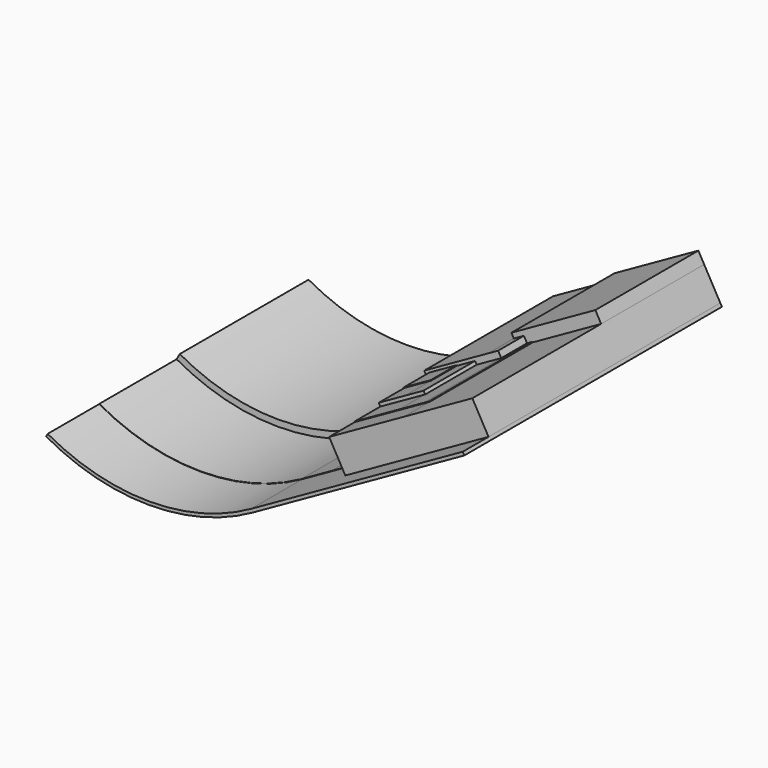
from build123d import *

# Parameters (mm, degrees)
F1_DEPTH = 100
F2_DEPTH = 90
F3_DEPTH = 80
F4_DEPTH = 80
F5_DEPTH = 70
F6_DEPTH = 60
F7_DEPTH = 50
F8_DEPTH = 40


with BuildPart() as f1:
    # F0 (on Front) → F1 (new body)
    with BuildSketch(Plane.XZ):
        with BuildLine():
            Line((50.8452397293, 26.2241268437), (29.5219979318, 14.223603626))
            ThreePointArc((29.5219979318, 14.223603626), (-2.0391196005, 5.9907088835), (-33.6008071966, 14.221417955))
            Line((-33.6008071966, 14.221417955), (-34.0891893351, 13.3487880868))
            ThreePointArc((-34.0891893351, 13.3487880868), (-2.0385061949, 4.9907089067), (30.0114505771, 13.3515729915))
            Line((30.0114505771, 13.3515729915), (95.813926037, 50.3845974272))
            Line((95.813926037, 50.3845974272), (95.3234723322, 51.2560646748))
            Line((95.3234723322, 51.2560646748), (50.8452397293, 26.2241268437))
        make_face()
    extrude(amount=F1_DEPTH)


with BuildPart() as f2:
    # F0 (on Front) → F2 (new body)
    with BuildSketch(Plane.XZ):
        Polygon((50.7948435843, 26.3136737049), (50.8452397293, 26.2241268437), (95.3234723322, 51.2560646748), (90.3044164077, 60.1742210862), (69.0536898036, 48.2145087485), (45.8261838048, 35.1422832552), (49.7882909537, 28.1021761505), align=None)
    extrude(amount=F2_DEPTH)


with BuildPart() as f3:
    # F0 (on Front) → F3 (new body)
    with BuildSketch(Plane.XZ):
        with BuildLine():
            ThreePointArc((-33.6008071966, 14.221417955), (-2.0391196005, 5.9907088835), (29.5219979318, 14.223603626))
            Line((29.5219979318, 14.223603626), (50.8452397293, 26.2241268437))
            Line((50.8452397293, 26.2241268437), (50.7948435843, 26.3136737049))
            Line((50.7948435843, 26.3136737049), (38.4987711206, 19.393557876))
            Line((38.4987711206, 19.393557876), (29.0659948309, 14.0848786448))
            ThreePointArc((29.0659948309, 14.0848786448), (-2.2719574378, 6.0911209367), (-33.5519689827, 14.3086809418))
            Line((-33.5519689827, 14.3086809418), (-33.6008071966, 14.221417955))
        make_face()
    extrude(amount=F3_DEPTH)


with BuildPart() as f4:
    # F0 (on Front) → F4 (new body)
    with BuildSketch(Plane.XZ):
        Polygon((45.8261838048, 35.1422832552), (69.0536898036, 48.2145087485), (68.9724342199, 48.3588884915), (67.2759677307, 47.4041328458), (59.6421667017, 43.1079002486), (45.7449282211, 35.2866629982), align=None)
    extrude(amount=F4_DEPTH)


with BuildPart() as f5:
    # F0 (on Front) → F5 (new body)
    with BuildSketch(Plane.XZ):
        Polygon((38.4987711206, 19.393557876), (50.7948435843, 26.3136737049), (49.7882909537, 28.1021761505), (43.2631740892, 24.5774321962), (37.4072678387, 21.4141830802), align=None)
    extrude(amount=F5_DEPTH)


with BuildPart() as f5b:
    # F0 (on Front) → F5, piece 2 (new body)
    with BuildSketch(Plane.XZ):
        Polygon((45.2470448009, 36.1713318051), (45.7449282211, 35.2866629982), (59.6421667017, 43.1079002486), (59.1442832815, 43.9925690556), (53.4865097086, 40.8084264301), align=None)
    extrude(amount=F5_DEPTH)


with BuildPart() as f6:
    # F0 (on Front) → F6 (new body)
    with BuildSketch(Plane.XZ):
        Polygon((43.2631740892, 24.5774321962), (49.7882909537, 28.1021761505), (45.8261838048, 35.1422832552), (45.7449282211, 35.2866629982), (45.2470448009, 36.1713318051), (53.4865097086, 40.8084264301), (53.4059276803, 40.95160936), (44.9516252368, 36.1936061575), (49.453318119, 28.1947311014), (43.1277044117, 24.8282179236), align=None)
    extrude(amount=F6_DEPTH)


with BuildPart() as f7:
    # F0 (on Front) → F7 (new body)
    with BuildSketch(Plane.XZ):
        with BuildLine():
            Line((-32.5752047057, 16.0539406781), (-33.5519689827, 14.3086809418))
            ThreePointArc((-33.5519689827, 14.3086809418), (-2.2719574378, 6.0911209367), (29.0659948309, 14.0848786448))
            Line((29.0659948309, 14.0848786448), (38.4987711206, 19.393557876))
            Line((38.4987711206, 19.393557876), (37.4072678387, 21.4141830802))
            Line((37.4072678387, 21.4141830802), (43.2631740892, 24.5774321962))
            Line((43.2631740892, 24.5774321962), (43.1277044117, 24.8282179236))
            Line((43.1277044117, 24.8282179236), (49.453318119, 28.1947311014))
            Line((49.453318119, 28.1947311014), (44.9516252368, 36.1936061575))
            Line((44.9516252368, 36.1936061575), (53.4059276803, 40.95160936))
            Line((53.4059276803, 40.95160936), (53.4865097086, 40.8084264301))
            Line((53.4865097086, 40.8084264301), (59.1442832815, 43.9925690556))
            Line((59.1442832815, 43.9925690556), (59.6421667017, 43.1079002486))
            Line((59.6421667017, 43.1079002486), (67.2759677307, 47.4041328458))
            Line((67.2759677307, 47.4041328458), (66.3095066613, 49.1213982263))
            Line((66.3095066613, 49.1213982263), (63.190689116, 47.3661565647))
            Line((63.190689116, 47.3661565647), (43.3571876206, 36.2040454072))
            Line((43.3571876206, 36.2040454072), (47.5722491088, 28.7144740215))
            Line((47.5722491088, 28.7144740215), (36.3952242818, 22.4241478499))
            Line((36.3952242818, 22.4241478499), (28.4962685386, 16.0560553203))
            ThreePointArc((28.4962685386, 16.0560553203), (-2.0391923145, 8.0907088823), (-32.5752047057, 16.0539406781))
        make_face()
    extrude(amount=F7_DEPTH)


with BuildPart() as f8:
    # F0 (on Front) → F8 (new body)
    with BuildSketch(Plane.XZ):
        Polygon((69.0536898036, 48.2145087485), (90.3044164077, 60.1742210862), (88.5034794178, 63.3742328025), (62.4374687791, 48.7045231575), (63.190689116, 47.3661565647), (66.3095066613, 49.1213982263), (67.2759677307, 47.4041328458), (68.9724342199, 48.3588884915), align=None)
    extrude(amount=F8_DEPTH)


solid = Compound([f1.part, f2.part, f3.part, f4.part, f5.part, f5b.part, f6.part, f7.part, f8.part])
